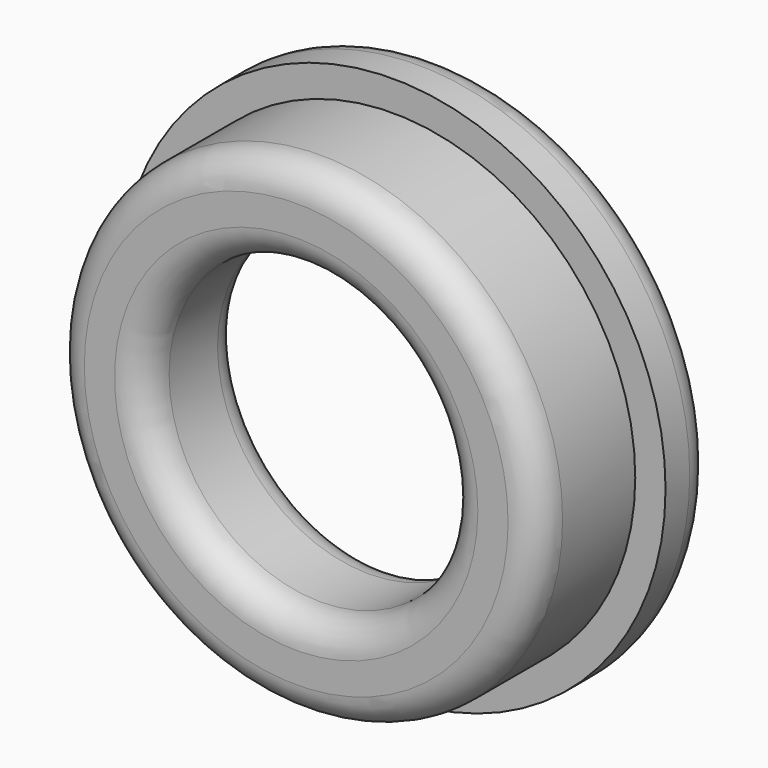
from build123d import *

# Parameters (mm, degrees)
F0_R     = 12.7
F0_R_2   = 7.9375
F1_DEPTH = 6.35
F0_R_3   = 14.2875
F2_DEPTH = 3.175
F3_R     = 1.58749
F3_2_R   = 1.58749


# Not quite as in the source:
# - a fillet or chamfer is up to 0.001 mm smaller than in the source, because OpenCascade refuses the exact size


with BuildPart() as f1:
    # F0 (on Front) → F1 (new body)
    with BuildSketch(Plane.XZ):
        Circle(F0_R)
        Circle(F0_R_2, mode=Mode.SUBTRACT)
    extrude(amount=F1_DEPTH)

    # F3 (radius 1.5875 in the source; OpenCascade refuses exactly that, so slightly less here)
    f3_edges = [f1.edges().sort_by_distance(p)[0] for p in [
        (-12.7, -6.35, 0),
        (-7.9375, -6.35, 0),
        (-7.9375, 0, 0),
    ]]
    fillet(f3_edges, radius=F3_R)


with BuildPart() as f2:
    # F0 (on Front) → F2 (new body)
    with BuildSketch(Plane.XZ):
        Circle(F0_R_3)
        Circle(F0_R, mode=Mode.SUBTRACT)
    extrude(amount=-F2_DEPTH)

    # F3#2 (radius 1.5875 in the source; OpenCascade refuses exactly that, so slightly less here)
    f3_2_edges = [f2.edges().sort_by_distance(p)[0] for p in [
        (-14.2875, 3.175, 0),
    ]]
    fillet(f3_2_edges, radius=F3_2_R)


solid = Compound([f1.part, f2.part])
